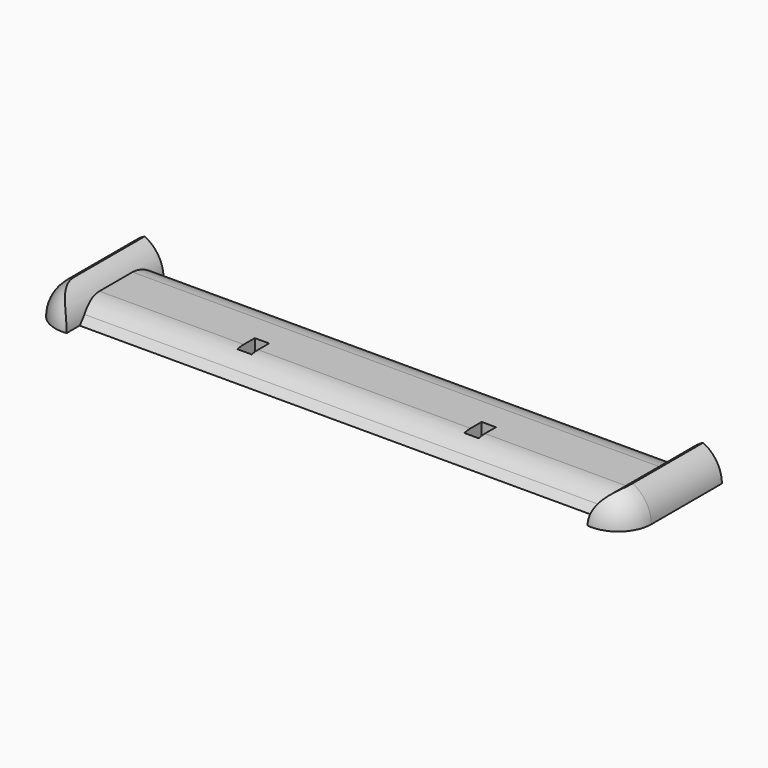
from build123d import *

# Parameters (mm, degrees)
F0_W          = 90
F0_H          = 18.32
F1_DEPTH      = 2.5
F2_W          = 2.16
F2_H          = 3.27
F3_DEPTH      = 25
F4_W          = 5
F4_H          = 18.32
F5_DEPTH      = 2.5
F6_T1_DEPTH   = 43.32
F6_T3_DEPTH   = 39.9706350946
F7_T1_DEPTH   = 39.9706350946
F7_T3_DEPTH   = 43.32
F8_T4_DEPTH   = 105.7168298797
F8_S5_R       = 5.0000000001
F8_T6_DEPTH   = 54
F8_S7_R       = 5.0000000001
F8_T8_DEPTH   = 54
F9_T4_DEPTH   = 105
F9_S5_R       = 5.0000000001
F9_T6_DEPTH   = 54
F9_S7_R       = 5.0000000001
F9_T8_DEPTH   = 54
F10_T4_ANGLE  = 350.8787991533
F10_S5_R      = 5.0000000001
F10_T6_DEPTH  = 9
F10_T10_ANGLE = 350.8787991654
F10_S11_R     = 5.0000000001
F10_T12_DEPTH = 9
F11_T4_DEPTH  = 90.3553390593
F11_S5_R      = 5.0000000001
F11_T6_DEPTH  = 47
F11_S7_R      = 5.0000000001
F11_T8_DEPTH  = 47


# Not quite as in the source:
# - a fillet or chamfer that OpenCascade refuses, or shapes differently, is made with other operations: its cross-section is extruded or revolved along the edge and cut away or added


with BuildPart() as f1:
    # F0 (on Top) → F1 (new body)
    with BuildSketch(Plane.XY):
        with Locations((28.5399998152, 34.3848172414)):
            Rectangle(F0_W, F0_H)
    extrude(amount=F1_DEPTH)

    # F2 (on face) → F3 (cut)
    with BuildSketch(Plane(origin=(0, 0, 0), x_dir=(1, 0, 0), z_dir=(0, 0, -1))):
        with Locations((11.4099998152, -32.7498172414)):
            Rectangle(F2_W, F2_H)
        with Locations((45.6699998152, -32.7498172414)):
            Rectangle(F2_W, F2_H)
    extrude(amount=-F3_DEPTH, mode=Mode.SUBTRACT)

    # F4 (on face) → F5 (join)
    with BuildSketch(Plane.XY.offset(2.5)):
        with Locations((-13.9600001848, 34.3848172414)):
            Rectangle(F4_W, F4_H)
        with Locations((71.0399998152, 34.3848172414)):
            Rectangle(F4_W, F4_H)
    extrude(amount=F5_DEPTH)

    # F6: fillet of radius 5 on 2 edges, made by hand

    # F6_s2 → F6_t1 (cut)
    with BuildSketch(Plane.XZ.offset(-56.0448172414)):
        with BuildLine():
            ThreePointArc((-16.4600001848, 0), (-14.9955340907, 3.5355339059), (-11.4600001848, 5))
            Line((-11.4600001848, 5), (-16.4600001848, 5))
            Line((-16.4600001848, 5), (-16.4600001848, 0))
        make_face()
    extrude(amount=F6_T1_DEPTH, mode=Mode.SUBTRACT)

    # F6_s4 → F6_t3 (cut)
    with BuildSketch(Plane.XZ.offset(-54.3701347887)):
        with BuildLine():
            ThreePointArc((-15.7901272037, 5), (-13.2901272037, 4.3301270189), (-11.4600001848, 2.5))
            Line((-11.4600001848, 2.5), (-11.4600001848, 5))
            Line((-11.4600001848, 5), (-15.7901272037, 5))
        make_face()
    extrude(amount=F6_T3_DEPTH, mode=Mode.SUBTRACT)

    # F7: fillet of radius 5 on 2 edges, made by hand

    # F7_s2 → F7_t1 (cut)
    with BuildSketch(Plane.XZ.offset(-54.3701347887)):
        with BuildLine():
            ThreePointArc((68.5399998152, 2.5), (70.3701268341, 4.3301270189), (72.8701268341, 5))
            Line((72.8701268341, 5), (68.5399998152, 5))
            Line((68.5399998152, 5), (68.5399998152, 2.5))
        make_face()
    extrude(amount=F7_T1_DEPTH, mode=Mode.SUBTRACT)

    # F7_s4 → F7_t3 (cut)
    with BuildSketch(Plane.XZ.offset(-56.0448172414)):
        with BuildLine():
            ThreePointArc((73.5399998152, 0), (72.0755337212, 3.5355339059), (68.5399998152, 5))
            Line((68.5399998152, 5), (73.5399998152, 5))
            Line((73.5399998152, 5), (73.5399998152, 0))
        make_face()
    extrude(amount=F7_T3_DEPTH, mode=Mode.SUBTRACT)

    # F8: chamfer of 5 on 1 edges, made by hand


with BuildPart() as f8_tool2:
    # F8_s3 → F8_t4 (new body)
    with BuildSketch(Plane.YZ.offset(-24.3184151246)):
        Polygon((30.2248172414, 2.5), (25.2248172414, -2.5), (25.2248172414, 2.5), align=None)
    extrude(amount=F8_T4_DEPTH)

    # F8_s5 → F8_t6 (cut, symmetric)
    with BuildSketch(Plane.XZ.offset(-27.7)):
        with Locations((-15.7901272038, -1e-10)):
            Circle(F8_S5_R)
    extrude(amount=F8_T6_DEPTH, both=True, mode=Mode.SUBTRACT)

    # F8_s7 → F8_t8 (cut, symmetric)
    with BuildSketch(Plane.XZ.offset(-27.7)):
        with Locations((72.8701268342, -1e-10)):
            Circle(F8_S7_R)
    extrude(amount=F8_T8_DEPTH, both=True, mode=Mode.SUBTRACT)


with BuildPart() as f1_1:
    add(f1.part)

    # F8_t1: cut F8_tool2
    add(f8_tool2.part, mode=Mode.SUBTRACT)

    # F9: fillet of radius 5 on 1 edges, made by hand


with BuildPart() as f9_tool2:
    # F9_s3 → F9_t4 (new body)
    with BuildSketch(Plane.YZ.offset(81.0399998152)):
        with BuildLine():
            ThreePointArc((43.5448172414, -2.5), (42.0803511473, 1.0355339059), (38.5448172414, 2.5))
            Line((38.5448172414, 2.5), (43.5448172414, 2.5))
            Line((43.5448172414, 2.5), (43.5448172414, -2.5))
        make_face()
    extrude(amount=-F9_T4_DEPTH)

    # F9_s5 → F9_t6 (cut, symmetric)
    with BuildSketch(Plane.XZ.offset(-41)):
        with Locations((72.8701268342, -1e-10)):
            Circle(F9_S5_R)
    extrude(amount=F9_T6_DEPTH, both=True, mode=Mode.SUBTRACT)

    # F9_s7 → F9_t8 (cut, symmetric)
    with BuildSketch(Plane.XZ.offset(-41)):
        with Locations((-15.7901272038, -1e-10)):
            Circle(F9_S7_R)
    extrude(amount=F9_T8_DEPTH, both=True, mode=Mode.SUBTRACT)


with BuildPart() as f1_2:
    add(f1_1.part)

    # F9_t1: cut F9_tool2
    add(f9_tool2.part, mode=Mode.SUBTRACT)

    # F10: fillet of radius 5 on 2 edges, made by hand


with BuildPart() as f10_tool2:
    # F10_s3 → F10_t4 (revolve)
    with BuildSketch(Plane(origin=(-4.0989769567, 0, -5.492965009), x_dir=(0, 1, 0), z_dir=(0.5980609221, 0, 0.8014506432))):
        with BuildLine():
            ThreePointArc((25.2248172414, 9.1846245187), (26.6892833355, 5.6490906128), (30.2248172414, 4.1846245187))
            Line((30.2248172414, 4.1846245187), (25.2248172414, 4.1846245187))
            Line((25.2248172414, 4.1846245187), (25.2248172414, 9.1846245187))
        make_face()
    revolve(axis=Axis((-11.4600001847, 25.2248172414, -1e-10), (0, 1, 0)), revolution_arc=F10_T4_ANGLE)

    # F10_s5 → F10_t6 (intersect, symmetric)
    with BuildSketch(Plane.XZ.offset(-27.7)):
        with Locations((-15.7901272038, -1e-10)):
            Circle(F10_S5_R)
    extrude(amount=F10_T6_DEPTH, both=True, mode=Mode.INTERSECT)


with BuildPart() as f1_3:
    add(f1_2.part)

    # F10_t1: cut F10_tool2
    add(f10_tool2.part, mode=Mode.SUBTRACT)


with BuildPart() as f10_tool8:
    # F10_s9 → F10_t10 (revolve)
    with BuildSketch(Plane(origin=(14.7214175546, 0, -28.147572216), x_dir=(0, 1, 0), z_dir=(0.4634498715, 0, -0.8861231385))):
        with BuildLine():
            ThreePointArc((25.2248172414, 60.7348797497), (26.6892833355, 57.1993458438), (30.2248172414, 55.7348797497))
            Line((30.2248172414, 55.7348797497), (25.2248172414, 55.7348797497))
            Line((25.2248172414, 55.7348797497), (25.2248172414, 60.7348797497))
        make_face()
    revolve(axis=Axis((68.5399998153, 25.2248172414, 1e-10), (0, 1, 0)), revolution_arc=F10_T10_ANGLE)

    # F10_s11 → F10_t12 (intersect, symmetric)
    with BuildSketch(Plane.XZ.offset(-27.7)):
        with Locations((72.8701268342, -1e-10)):
            Circle(F10_S11_R)
    extrude(amount=F10_T12_DEPTH, both=True, mode=Mode.INTERSECT)


with BuildPart() as f1_4:
    add(f1_3.part)

    # F10_t7: cut F10_tool8
    add(f10_tool8.part, mode=Mode.SUBTRACT)

    # F11: fillet of radius 5 on 1 edges, made by hand


with BuildPart() as f11_tool2:
    # F11_s3 → F11_t4 (new body)
    with BuildSketch(Plane.YZ.offset(-16.6376697145)):
        with BuildLine():
            ThreePointArc((28.7603511473, 1.0355339059), (30.3824678914, 2.1193976626), (32.2958850533, 2.5))
            Line((32.2958850533, 2.5), (30.2248172414, 2.5))
            Line((30.2248172414, 2.5), (28.7603511473, 1.0355339059))
        make_face()
    extrude(amount=F11_T4_DEPTH)

    # F11_s5 → F11_t6 (cut, symmetric)
    with BuildSketch(Plane.XZ.offset(-30.5)):
        with Locations((72.8701268342, -1e-10)):
            Circle(F11_S5_R)
    extrude(amount=F11_T6_DEPTH, both=True, mode=Mode.SUBTRACT)

    # F11_s7 → F11_t8 (cut, symmetric)
    with BuildSketch(Plane.XZ.offset(-30.5)):
        with Locations((-15.7901272038, -1e-10)):
            Circle(F11_S7_R)
    extrude(amount=F11_T8_DEPTH, both=True, mode=Mode.SUBTRACT)


with BuildPart() as f1_5:
    add(f1_4.part)

    # F11_t1: cut F11_tool2
    add(f11_tool2.part, mode=Mode.SUBTRACT)


solid = f1_5.part
